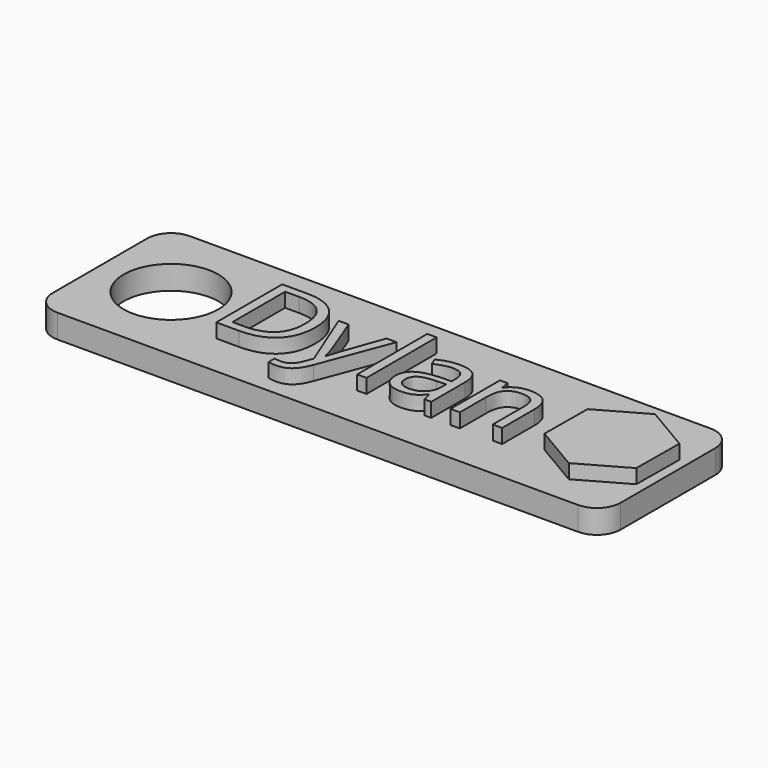
from build123d import *

# Parameters (mm, degrees)
F0_W         = 120
F0_H         = 35
F0_R         = 10
F1_DEPTH     = 5
F2_R         = 5
F3_TEXT_SIZE = 24.3778495739
F4_DEPTH     = 3
F6_DEPTH     = 3


# Not quite as in the source:
# - Text() gives the source's letters only with a copy of the font that has no kerning and outlines rounded to 1/6400 em; it was checked with that copy


with BuildPart() as f1:
    # F0 (on Top) → F1 (new body)
    with BuildSketch(Plane.XY):
        Rectangle(F0_W, F0_H)
        with Locations((-45, 0)):
            Circle(F0_R, mode=Mode.SUBTRACT)
    extrude(amount=F1_DEPTH)

    # F2
    f2_edges = [f1.edges().sort_by_distance(p)[0] for p in [
        (-60, 17.5, 2.5),
        (-60, -17.5, 2.5),
        (60, -17.5, 2.5),
        (60, 17.5, 2.5),
    ]]
    fillet(f2_edges, radius=F2_R)

    # F3 (on face) → F4 (join)
    with BuildSketch(Plane.XY.offset(5)):
        with Locations((-31.1548896134, -8.3372183144)):
            Text('Dylan', F3_TEXT_SIZE, font='Open Sans', text_align=(TextAlign.LEFT, TextAlign.BOTTOM))
    extrude(amount=F4_DEPTH)

    # F5 (on face) → F6 (join)
    with BuildSketch(Plane.XY.offset(5)):
        Polygon((48.2472669894, 11.2785175325), (38.43438955, 5.717884761), (38.3436000716, -5.5606327715), (48.0656880325, -11.2785175325), (57.8785654718, -5.717884761), (57.9693549503, 5.5606327715), align=None)
    extrude(amount=F6_DEPTH)


solid = f1.part
